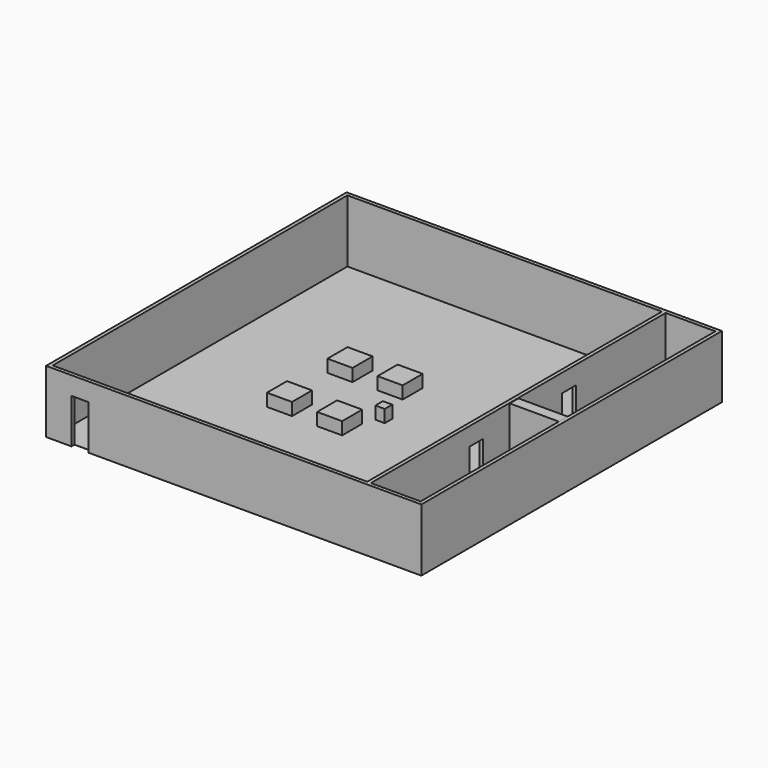
from build123d import *

# Parameters (mm, degrees)
F1_DEPTH      = 0.0254
F2_W          = 1.4732
F2_H          = 1.4732
F2_W_2        = 149.2444640862
F2_H_2        = 149.4354150163
F3_DEPTH      = 25.4
F4_W          = 7.000075886
F4_H          = 18.0553272367
F5_DEPTH      = 1.524
F6_W          = 10.16
F6_H          = 10.16
F6_W_2        = 3.81
F6_H_2        = 3.81
F7_DEPTH      = 5.08
F10_DEPTH     = 149.86
F11_DEPTH     = 0.508
F12_W         = 7.0104
F12_H         = 18.0594
F13_DEPTH     = 12.7
F14_W         = 4.4178627431
F14_H         = 25.2445153892
F15_DEPTH     = 20.5232
F17_DEPTH     = 2.3114
F18_TEXT_SIZE = 11.0697777321
F19_DEPTH     = 0.254
F20_TEXT_SIZE = 7.4287035709
F21_DEPTH     = 0.254


# Not quite as in the source:
# - Text() gives the source's letters only with a copy of the font that has no kerning and outlines rounded to 1/6400 em; it was checked with that copy


with BuildPart() as f1:
    # F0 (on Top) → F1 (new body)
    with BuildSketch(Plane.XY):
        Polygon((76.2502923608, 76.0954320431), (0, 76.0954320431), (-75.9405717254, 76.0954320431), (-75.9405717254, 0), (-75.9405717254, -76.2863829732), (76.2502923608, -76.2863829732), (76.2502923608, 0), align=None)
    extrude(amount=F1_DEPTH)

    # F2 (on face) → F3 (join)
    with BuildSketch(Plane.XY.offset(0.0254)):
        with Locations((-75.2039717254, 75.3588320431)):
            Rectangle(F2_W, F2_H)
        Polygon((-74.4673717254, 74.6222320431), (-75.9405717254, 74.6222320431), (-75.9405717254, -76.2863829732), (-74.4673717254, -76.2863829732), (-74.4673717254, -74.8131829732), align=None)
        with Locations((0.1548603177, 75.3588320431)):
            Rectangle(F2_W_2, F2_H)
        with Locations((75.5136923608, 75.3588320431)):
            Rectangle(F2_W, F2_H)
        with Locations((0.1548603177, -75.5497829732)):
            Rectangle(F2_W_2, F2_H)
        with Locations((75.5136923608, -0.0954754651)):
            Rectangle(F2_W, F2_H_2)
        with Locations((75.5136923608, -75.5497829732)):
            Rectangle(F2_W, F2_H)
    extrude(amount=F3_DEPTH)

    # F4 (on face) → F5 (cut)
    with BuildSketch(Plane.XZ.offset(76.2863829732)):
        with Locations((-62.1423841221, 9.0276636183)):
            Rectangle(F4_W, F4_H)
    extrude(amount=-F5_DEPTH, mode=Mode.SUBTRACT)

    # F6 (on face) → F7 (join)
    with BuildSketch(Plane.XY.offset(0.0254)):
        with Locations((-8.8592786342, 19.3496923894)):
            Rectangle(F6_W, F6_H)
        Rectangle(F6_W_2, F6_H_2)
        with Locations((-8.4771532565, -11.7935594171)):
            Rectangle(F6_W, F6_H)
        with Locations((-28.7298187613, 18.7765043229)):
            Rectangle(F6_W, F6_H)
        with Locations((-29.1119460016, -11.4114331082)):
            Rectangle(F6_W, F6_H)
    extrude(amount=F7_DEPTH)

    # F9 (on face) → F10 (join)
    with BuildSketch(Plane(origin=(0, -74.8131829732, 0), x_dir=(-1, 0, 0), z_dir=(0, 1, 0))):
        Polygon((-54.5995202429, 25.4254), (-54.5995202429, 0.0254), (-53.1263202429, 0), (-53.1263202429, 25.4254), align=None)
    extrude(amount=F10_DEPTH)

    # F9 (on face) → F11 (join)
    with BuildSketch(Plane(origin=(0, -74.8131829732, 0), x_dir=(-1, 0, 0), z_dir=(0, 1, 0))):
        Polygon((-54.5995202429, 25.4254), (-54.5995202429, 0.0254), (-53.1263202429, 0), (-53.1263202429, 25.4254), align=None)
    extrude(amount=-F11_DEPTH)

    # F12 (on face) → F13 (cut)
    with BuildSketch(Plane(origin=(53.1263202429, 0, 0), x_dir=(0, -1, 0), z_dir=(-1, 0, 0))):
        with Locations((21.4227622761, 9.0551)):
            Rectangle(F12_W, F12_H)
        with Locations((-25.6271661804, 9.0551)):
            Rectangle(F12_W, F12_H)
    extrude(amount=-F13_DEPTH, mode=Mode.SUBTRACT)

    # F14 (on face) → F15 (join)
    with BuildSketch(Plane(origin=(74.7770923608, 0, 0), x_dir=(0, -1, 0), z_dir=(-1, 0, 0))):
        with Locations((2.2089313716, 12.6222576946)):
            Rectangle(F14_W, F14_H)
    extrude(amount=F15_DEPTH)

    # F16 (on face) → F17 (join)
    with BuildSketch(Plane(origin=(74.7770923608, 0, 0), x_dir=(0, -1, 0), z_dir=(-1, 0, 0))):
        Polygon((4.4296383858, 3.8450045977), (4.4296383858, 0), (25.3371190162, 0), (25.6655806558, 3.8450045977), align=None)
    extrude(amount=F17_DEPTH)

    # F18 (on face) → F19 (cut)
    with BuildSketch(Plane(origin=(53.1263202429, 0, 0), x_dir=(0, -1, 0), z_dir=(-1, 0, 0))):
        with Locations((29.1266478598, 11.12976484)):
            Text('Printers', F18_TEXT_SIZE, font='Open Sans', text_align=(TextAlign.LEFT, TextAlign.BOTTOM))
    extrude(amount=-F19_DEPTH, mode=Mode.SUBTRACT)

    # F20 (on face) → F21 (cut)
    with BuildSketch(Plane(origin=(53.1263202429, 0, 0), x_dir=(0, -1, 0), z_dir=(-1, 0, 0))):
        with Locations((-67.0333132148, 13.8709368184)):
            Text('Storage', F20_TEXT_SIZE, font='Open Sans', text_align=(TextAlign.LEFT, TextAlign.BOTTOM))
    extrude(amount=-F21_DEPTH, mode=Mode.SUBTRACT)


solid = f1.part
